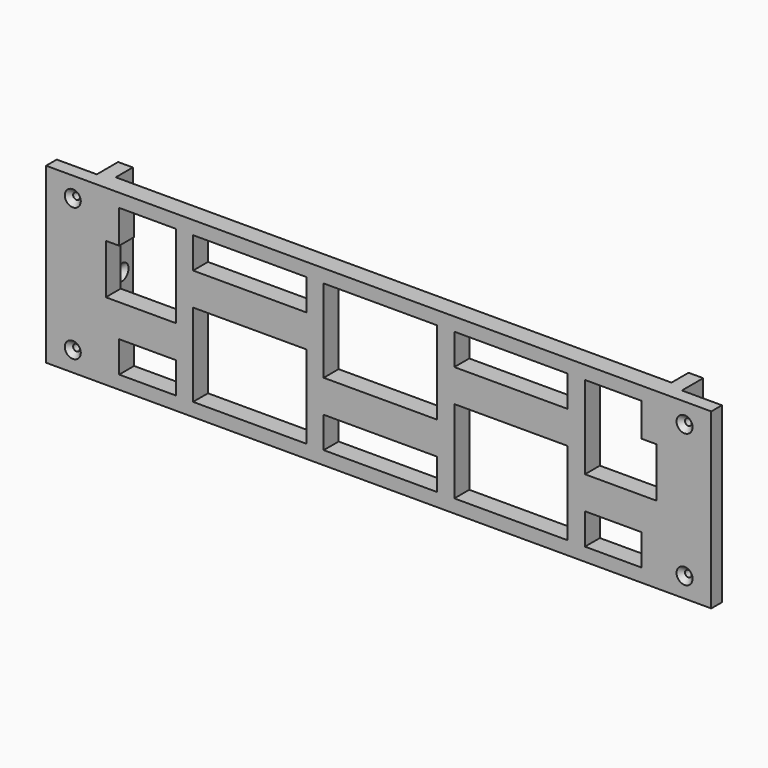
from build123d import *

# Parameters (mm, degrees)
F0_W      = 438.5
F0_H      = 130
F1_DEPTH  = 14
F2_W      = 30
F2_H      = 10
F3_DEPTH  = 130
F4_W      = 11
F4_H      = 16
F5_DEPTH  = 130
F6_W      = 42.5
F6_H      = 23.3528089888
F6_H_2    = 62.2471910113
F7_DEPTH  = 25
F8_R      = 2.5
F9_DEPTH  = 25
F10_R     = 2.5
F11_DEPTH = 468.501
F12_SIZE  = 3.49999


# Not quite as in the source:
# - a fillet or chamfer is up to 0.001 mm smaller than in the source, because OpenCascade refuses the exact size
# - a feature names something its author has since deleted; it is built from what else it names


with BuildPart() as f1:
    # F0 (on Front) → F1 (new body)
    with BuildSketch(Plane.XZ):
        with Locations((219.25, 65)):
            Rectangle(F0_W, F0_H)
    extrude(amount=F1_DEPTH)

    # F2 (on face) → F3 (join, through all)
    with BuildSketch(Plane.XY.offset(130)):
        with Locations((453.5, -9)):
            Rectangle(F2_W, F2_H)
        with Locations((-15, -9)):
            Rectangle(F2_W, F2_H)
    extrude(amount=-F3_DEPTH)

    # F4 (on face) → F5 (join, through all)
    with BuildSketch(Plane.XY.offset(130)):
        with Locations((5.5, 8)):
            Rectangle(F4_W, F4_H)
        with Locations((433, 8)):
            Rectangle(F4_W, F4_H)
    extrude(amount=-F5_DEPTH)

    # F6 (on face) → F7 (cut)
    with BuildSketch(Plane.XZ.offset(14)):
        Polygon((24.75, 120), (24.75, 95), (14.75, 95), (14.75, 57.7528089887), (24.75, 57.7528089887), (67.25, 57.7528089887), (67.25, 120), align=None)
        with Locations((46, 21.6764044942)):
            Rectangle(F6_W, F6_H)
        with Locations((101.4, 41.1235955055)):
            Rectangle(F6_W, F6_H_2)
        with Locations((143.9, 41.1235955055)):
            Rectangle(F6_W, F6_H_2)
        with Locations((101.4, 108.3235955056)):
            Rectangle(F6_W, F6_H)
        with Locations((143.9, 108.3235955056)):
            Rectangle(F6_W, F6_H)
        with Locations((199.3, 88.8764044943)):
            Rectangle(F6_W, F6_H_2)
        with Locations((241.8, 88.8764044943)):
            Rectangle(F6_W, F6_H_2)
        with Locations((199.3, 21.6764044942)):
            Rectangle(F6_W, F6_H)
        with Locations((241.8, 21.6764044942)):
            Rectangle(F6_W, F6_H)
        with Locations((297.2, 41.1235955055)):
            Rectangle(F6_W, F6_H_2)
        with Locations((339.7, 41.1235955055)):
            Rectangle(F6_W, F6_H_2)
        with Locations((339.7, 108.3235955056)):
            Rectangle(F6_W, F6_H)
        with Locations((297.2, 108.3235955056)):
            Rectangle(F6_W, F6_H)
        Polygon((416.35, 120), (373.85, 120), (373.85, 57.7528089887), (427.35, 57.7528089887), (427.35, 95), (416.35, 95), align=None)
        with Locations((395.1, 21.6764044942)):
            Rectangle(F6_W, F6_H)
    extrude(amount=-F7_DEPTH, mode=Mode.SUBTRACT)

    # F8 (on face) → F9 (cut)
    with BuildSketch(Plane(origin=(0, -4, 0), x_dir=(-1, 0, 0), z_dir=(0, 1, 0))):
        with Locations((-448.5, 115)):
            Circle(F8_R)
        with Locations((-448.5, 15)):
            Circle(F8_R)
        with Locations((10, 115)):
            Circle(F8_R)
        with Locations((10, 15)):
            Circle(F8_R)
    extrude(amount=-F9_DEPTH, mode=Mode.SUBTRACT)

    # F10 (on face) → F11 (cut, through all)
    with BuildSketch(Plane.YZ.offset(438.5)):
        with Locations((6, 115)):
            Circle(F10_R)
        with Locations((6, 15)):
            Circle(F10_R)
        with Locations((6, 65)):
            Circle(F10_R)
    extrude(amount=-F11_DEPTH, mode=Mode.SUBTRACT)

    # F12 (size 3.5 in the source; OpenCascade refuses exactly that, so slightly less here)
    f12_edges = [f1.edges().sort_by_distance(p)[0] for p in [
        (451, -14, 115),
        (451, -14, 15),
        (-7.5, -14, 115),
        (-7.5, -14, 15),
        (427.5, 3.5, 115),
        (427.5, 3.5, 65),
        (427.5, 3.5, 15),
        (11, 3.5, 115),
        (11, 3.5, 65),
        (11, 3.5, 15),
    ]]
    chamfer(f12_edges, length=F12_SIZE)


solid = f1.part
